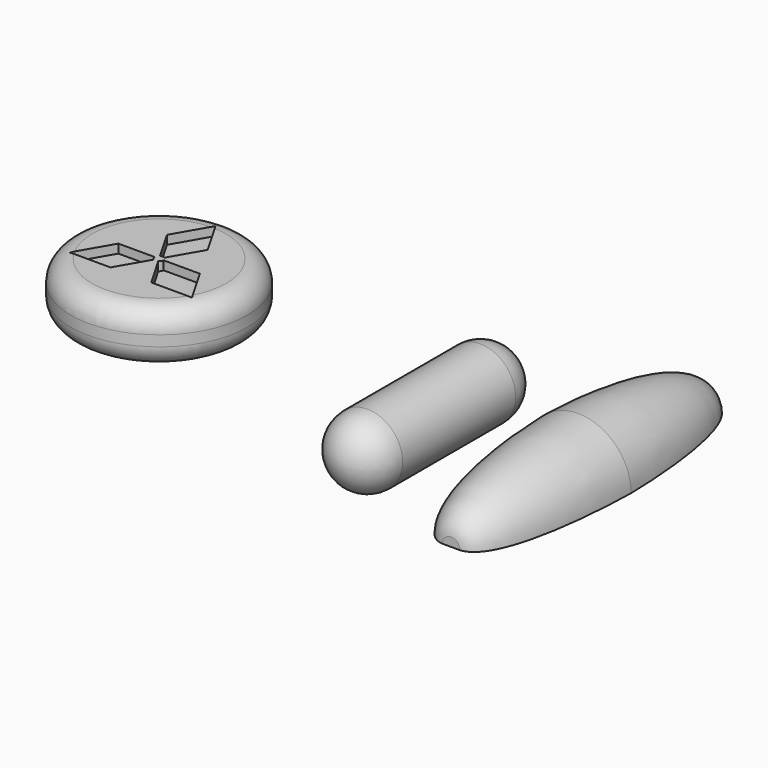
from build123d import *

# Parameters (mm, degrees)
F2_R     = 5
F3_DEPTH = 3
F4_START = 0.5
F4_DEPTH = 2
F7_ANGLE = 180


# Not quite as in the source:
# - a fillet or chamfer that OpenCascade refuses, or shapes differently, is made with other operations: its cross-section is extruded or revolved along the edge and cut away or added


with BuildPart() as f1:
    # F0 (on Top) → F1 (revolve)
    with BuildSketch(Plane.XY):
        with BuildLine():
            Line((0, 6), (0, 0))
            Line((0, 0), (0, -6))
            ThreePointArc((0, -6), (1.4142135624, -5.4142135624), (2, -4))
            Line((2, -4), (2, 4))
            ThreePointArc((2, 4), (1.4142135624, 5.4142135624), (0, 6))
        make_face()
    revolve(axis=Axis((0, 3, 0), (0, 1, 0)))


with BuildPart() as f3:
    # F2 (on Top) → F3 (new body)
    with BuildSketch(Plane.XY):
        with Locations((-15, 0)):
            Circle(F2_R)
        with BuildLine():
            Line((-16.1547005384, 2), (-15, 4))
            Line((-15, 4), (-13.8452994616, 2))
            Line((-13.8452994616, 2), (-14.875, 0.2165063509))
            ThreePointArc((-14.875, 0.2165063509), (-14.7834936491, 0.125), (-14.75, 0))
            Line((-14.75, 0), (-12.6905989232, 0))
            Line((-12.6905989232, 0), (-11.5358983849, -2))
            Line((-11.5358983849, -2), (-13.8452994616, -2))
            Line((-13.8452994616, -2), (-14.875, -0.2165063509))
            ThreePointArc((-14.875, -0.2165063509), (-15, -0.25), (-15.125, -0.2165063509))
            Line((-15.125, -0.2165063509), (-16.1547005384, -2))
            Line((-16.1547005384, -2), (-18.4641016151, -2))
            Line((-18.4641016151, -2), (-17.3094010768, 0))
            Line((-17.3094010768, 0), (-15.25, 0))
            ThreePointArc((-15.25, 0), (-15.2165063509, 0.125), (-15.125, 0.2165063509))
            Line((-15.125, 0.2165063509), (-16.1547005384, 2))
        make_face(mode=Mode.SUBTRACT)
        with BuildLine():
            ThreePointArc((-14.875, 0.2165063509), (-15, 0.25), (-15.125, 0.2165063509))
            ThreePointArc((-15.125, 0.2165063509), (-15.2165063509, 0.125), (-15.25, 0))
            ThreePointArc((-15.25, 0), (-15.2165063509, -0.125), (-15.125, -0.2165063509))
            ThreePointArc((-15.125, -0.2165063509), (-15, -0.25), (-14.875, -0.2165063509))
            ThreePointArc((-14.875, -0.2165063509), (-14.7834936491, -0.125), (-14.75, 0))
            ThreePointArc((-14.75, 0), (-14.7834936491, 0.125), (-14.875, 0.2165063509))
        make_face()
    extrude(amount=F3_DEPTH)

    # F2 (on Top) → F4 (join)
    with BuildSketch(Plane.XY.offset(F4_START)):
        with BuildLine():
            ThreePointArc((-15.125, -0.2165063509), (-15.2165063509, -0.125), (-15.25, 0))
            Line((-15.25, 0), (-17.3094010768, 0))
            Line((-17.3094010768, 0), (-18.4641016151, -2))
            Line((-18.4641016151, -2), (-16.1547005384, -2))
            Line((-16.1547005384, -2), (-15.125, -0.2165063509))
        make_face()
        with BuildLine():
            Line((-12.6905989232, 0), (-14.75, 0))
            ThreePointArc((-14.75, 0), (-14.7834936491, -0.125), (-14.875, -0.2165063509))
            Line((-14.875, -0.2165063509), (-13.8452994616, -2))
            Line((-13.8452994616, -2), (-11.5358983849, -2))
            Line((-11.5358983849, -2), (-12.6905989232, 0))
        make_face()
        with BuildLine():
            Line((-13.8452994616, 2), (-15, 4))
            Line((-15, 4), (-16.1547005384, 2))
            Line((-16.1547005384, 2), (-15.125, 0.2165063509))
            ThreePointArc((-15.125, 0.2165063509), (-15, 0.25), (-14.875, 0.2165063509))
            Line((-14.875, 0.2165063509), (-13.8452994616, 2))
        make_face()
    extrude(amount=F4_DEPTH)

    # F5: fillet of radius 1.2 on 3 edges, made by hand

    # F5_s1 → F5_t2 (revolve, cut)
    with BuildSketch(Plane.XZ):
        with BuildLine():
            ThreePointArc((-10, 1.2), (-10.3514718626, 0.3514718626), (-11.2, 0))
            Line((-11.2, 0), (-10, 0))
            Line((-10, 0), (-10, 1.2))
        make_face()
    revolve(axis=Axis((-15, 0, 0), (0, 0, 1)), mode=Mode.SUBTRACT)

    # F5_s3 → F5_t4 (revolve, cut)
    with BuildSketch(Plane.XZ):
        with BuildLine():
            ThreePointArc((-10, 1.8), (-10.3514718626, 2.6485281374), (-11.2, 3))
            Line((-11.2, 3), (-10, 3))
            Line((-10, 3), (-10, 1.8))
        make_face()
    revolve(axis=Axis((-15, 0, 3), (0, 0, 1)), mode=Mode.SUBTRACT)


with BuildPart() as f7:
    # F6 (on Top) → F7 (revolve)
    with BuildSketch(Plane.XY):
        with BuildLine():
            Line((8.7468870582, 9), (8.7468870582, 0))
            Line((8.7468870582, 0), (8.7468870582, -9))
            Line((8.7468870582, -9), (9.2468870582, -9))
            add(Edge.make_bspline(
                [(9.2468870582, -9), (11.1883362318, -8.8468901743), (11.6957966082, -2.9714520147), (11.7468870582, 0)],
                knots=[0, 0, 0, 0, 9.3407708461, 9.3407708461, 9.3407708461, 9.3407708461], degree=3))
            add(Edge.make_bspline(
                [(9.2468870582, 9), (11.1883362318, 8.8468901743), (11.6957966082, 2.9714520147), (11.7468870582, 0)],
                knots=[0, 0, 0, 0, 9.3407708461, 9.3407708461, 9.3407708461, 9.3407708461], degree=3))
            Line((9.2468870582, 9), (8.7468870582, 9))
        make_face()
    revolve(axis=Axis((8.7468870582, 4.5, 0), (0, -1, 0)), revolution_arc=F7_ANGLE)


solid = Compound([f1.part, f3.part, f7.part])
